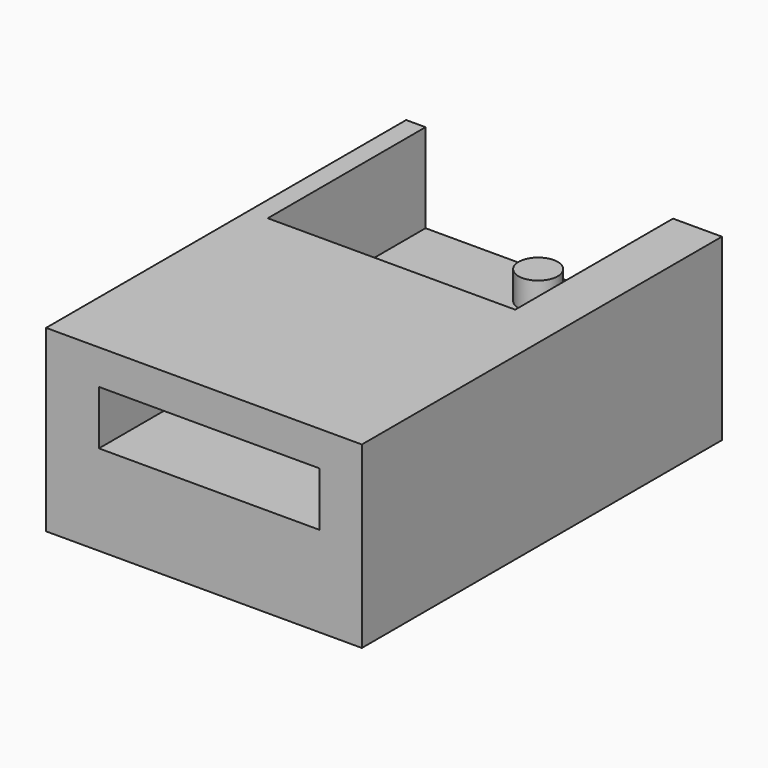
from build123d import *

# Parameters (mm, degrees)
F0_W     = 71.2816417217
F0_H     = 40.4414199293
F2_DEPTH = 101.6
F1_W     = 49.7516710311
F1_H     = 12.2197093442
F3_DEPTH = 101.6
F4_R     = 4.4126696885
F5_DEPTH = 6.35
F6_W     = 55.8680891991
F6_H     = 44.7704729486
F7_DEPTH = 101.6
F8_DEPTH = 6.35


with BuildPart() as f2:
    # F0 (on Front) → F2 (new body)
    with BuildSketch(Plane.XZ):
        with Locations((-1.6001984477, -0.1454725862)):
            Rectangle(F0_W, F0_H)
    extrude(amount=F2_DEPTH)

    # F1 (on Front) → F3 (cut)
    with BuildSketch(Plane.XZ):
        with Locations((-0.4364186898, 6.1098546721)):
            Rectangle(F1_W, F1_H)
    extrude(amount=F3_DEPTH, mode=Mode.SUBTRACT)

    # F4 (on Top) → F5 (join)
    with BuildSketch(Plane.XY):
        with Locations((0, -9.3056354672)):
            Circle(F4_R)
    extrude(amount=F5_DEPTH)

    # F6 (on Top) → F7 (cut)
    with BuildSketch(Plane.XY):
        with Locations((-4.929035902, -22.1368068433)):
            Rectangle(F6_W, F6_H)
    extrude(amount=F7_DEPTH, mode=Mode.SUBTRACT)

    # F4 (on Top) → F8 (join)
    with BuildSketch(Plane.XY):
        with Locations((0, -9.3056354672)):
            Circle(F4_R)
    extrude(amount=F8_DEPTH)


solid = f2.part
